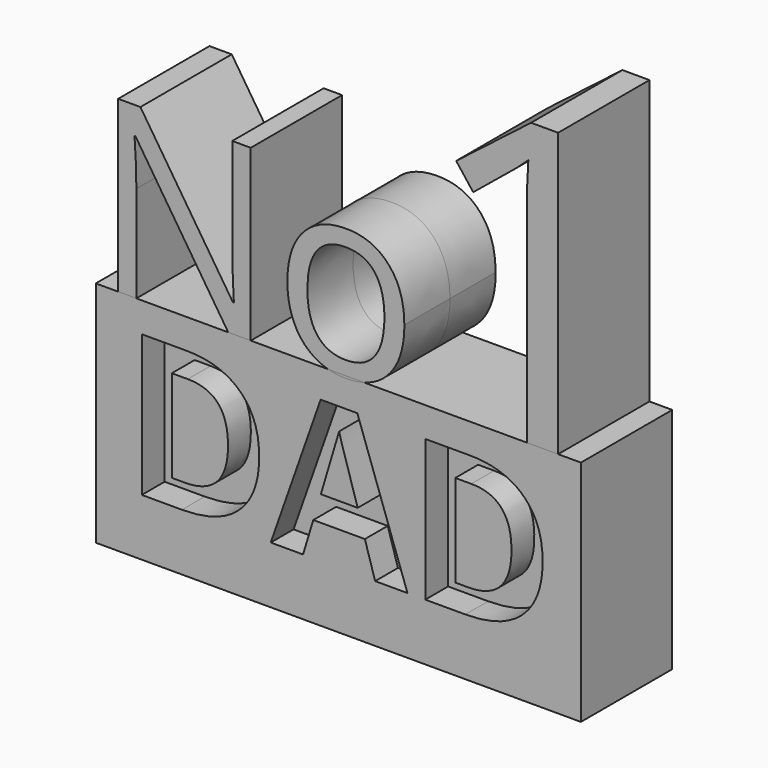
from build123d import *

# Parameters (mm, degrees)
F0_TEXT_SIZE   = 41.6666666667
F0_TEXT_SIZE_2 = 69.4444444444
F1_DEPTH       = 10
F2_W           = 85
F2_H           = 40
F3_DEPTH       = 10
F4_TEXT_SIZE   = 34.7222222222
F5_DEPTH       = 5


# Not quite as in the source:
# - Text() gives the source's letters only with a copy of the font that has no kerning and outlines rounded to 1/6400 em; it was checked with that copy


with BuildPart() as f1:
    # F0 (on Front) → F1 (new body, symmetric)
    with BuildSketch(Plane.XZ):
        with Locations((-56.9401041667, 0)):
            Text('No', F0_TEXT_SIZE, font='Open Sans', text_align=(TextAlign.LEFT, TextAlign.BOTTOM))
        with Locations((0, 0)):
            Text('1', F0_TEXT_SIZE_2, font='Open Sans', text_align=(TextAlign.LEFT, TextAlign.BOTTOM))
    extrude(amount=F1_DEPTH, both=True)

    # F2 (on Front) → F3 (join, symmetric)
    with BuildSketch(Plane.XZ):
        with Locations((-14.2670240998, -20)):
            Rectangle(F2_W, F2_H)
    extrude(amount=F3_DEPTH, both=True)

    # F4 (on face) → F5 (cut)
    with BuildSketch(Plane.XZ.offset(10)):
        with Locations((-51.8205963135, -30.0057576248)):
            Text('DAD', F4_TEXT_SIZE, font='Open Sans', font_style=FontStyle.BOLD, text_align=(TextAlign.LEFT, TextAlign.BOTTOM))
    extrude(amount=-F5_DEPTH, mode=Mode.SUBTRACT)


solid = f1.part
